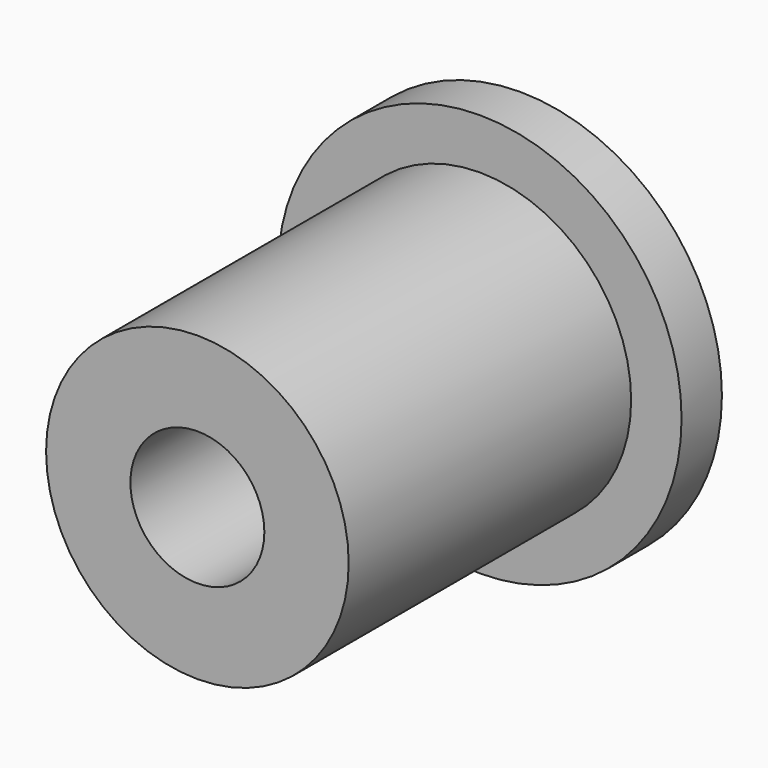
from build123d import *

# Parameters (mm, degrees)
F0_R     = 12.7
F0_R_2   = 4.2164
F1_DEPTH = 25.4
F2_R     = 12.7
F2_R_2   = 9.525
F3_DEPTH = 22.225


# Not quite as in the source:
# - a length typed as a fraction of an inch, garbled in the dataset ("3 / 203.2 mm" for 3/8 in), is restored


with BuildPart() as f1:
    # F0 (on Front) → F1 (new body)
    with BuildSketch(Plane.XZ):
        Circle(F0_R)
        Circle(F0_R_2, mode=Mode.SUBTRACT)
    extrude(amount=F1_DEPTH)

    # F2 (on face) → F3 (cut)
    with BuildSketch(Plane.XZ.offset(25.4)):
        Circle(F2_R)
        Circle(F2_R_2, mode=Mode.SUBTRACT)
    extrude(amount=-F3_DEPTH, mode=Mode.SUBTRACT)


solid = f1.part
